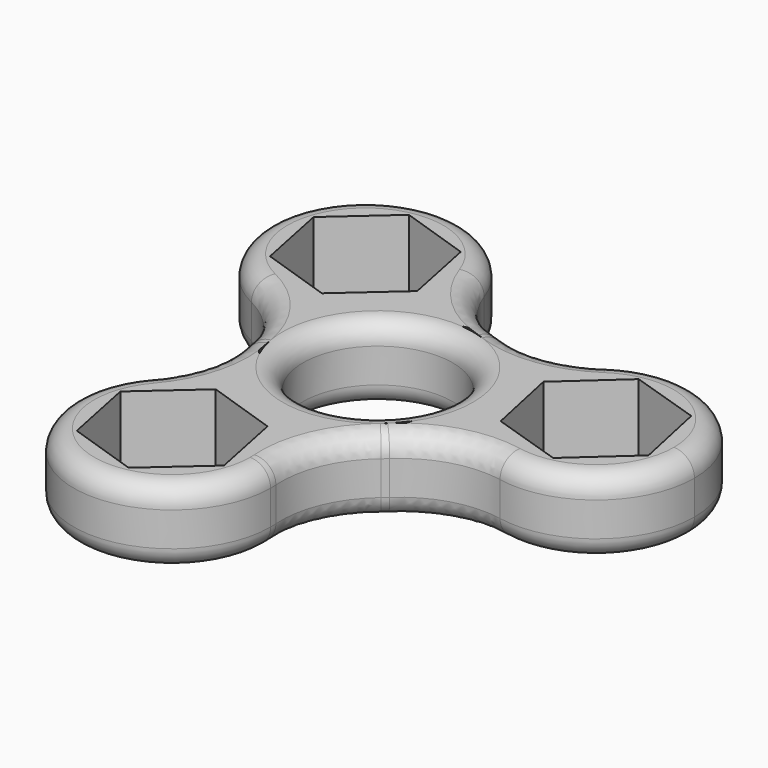
from build123d import *

# Parameters (mm, degrees)
F0_R     = 10.95
F1_DEPTH = 11
F2_R     = 15
F3_R     = 3
F4_R     = 3
F5_R     = 2.99999


# Not quite as in the source:
# - a fillet or chamfer is up to 0.001 mm smaller than in the source, because OpenCascade refuses the exact size


with BuildPart() as f1:
    # F0 (on Top) → F1 (new body)
    with BuildSketch(Plane.XY):
        with BuildLine():
            ThreePointArc((16.654712117, -4.1714415358), (16.9775112004, -2.2849104924), (17.0855701569, -0.3740149201))
            ThreePointArc((17.0855701569, -0.3740149201), (16.2517047433, 4.8769569892), (13.8321535207, 9.6112794751))
            ThreePointArc((13.8321535207, 9.6112794751), (13.447376375, 2.3521052012), (16.654712117, -4.1714415358))
        make_face()
        with BuildLine():
            ThreePointArc((13.8321535207, 9.6112794751), (16.2517047433, 4.8769569892), (17.0855701569, -0.3740149201))
            ThreePointArc((17.0855701569, -0.3740149201), (16.9775112004, -2.2849104924), (16.654712117, -4.1714415358))
            ThreePointArc((16.654712117, -4.1714415358), (32.5885679794, -8.2650064174), (41.9781924859, 5.2435089603))
            ThreePointArc((41.9781924859, 5.2435089603), (29.7762969315, 19.4849706892), (13.8321535207, 9.6112794751))
        make_face()
        Polygon((25.2852360408, 15.9143511546), (35.6669746396, 12.5543654899), (37.948010997, 1.8835232956), (29.8473087557, -5.4273332341), (19.4655701569, -2.0673475694), (17.1845337995, 8.6034946249), align=None, mode=Mode.SUBTRACT)
        with BuildLine():
            ThreePointArc((16.654712117, -4.1714415358), (13.447376375, 2.3521052012), (13.8321535207, 9.6112794751))
            ThreePointArc((13.8321535207, 9.6112794751), (5.4932428297, 15.7069627719), (-4.835332905, 15.8306949739))
            ThreePointArc((-4.835332905, 15.8306949739), (-8.8812222309, 9.7912873743), (-15.3602401355, 6.4949270203))
            ThreePointArc((-15.3602401355, 6.4949270203), (-16.4698013785, -3.7746231263), (-11.4126687413, -12.7812981985))
            ThreePointArc((-11.4126687413, -12.7812981985), (-4.1594436733, -13.2654373359), (1.9347970856, -17.2282512558))
            ThreePointArc((1.9347970856, -17.2282512558), (11.3832690194, -13.054384406), (16.654712117, -4.1714415358))
        make_face()
        with Locations((0.1355701569, -0.3740149201)):
            Circle(F0_R, mode=Mode.SUBTRACT)
        with BuildLine():
            ThreePointArc((-15.3602401355, 6.4949270203), (-8.8812222309, 9.7912873743), (-4.835332905, 15.8306949739))
            ThreePointArc((-4.835332905, 15.8306949739), (-11.1121287057, 12.3063545657), (-15.3602401355, 6.4949270203))
        make_face()
        with BuildLine():
            ThreePointArc((-15.3602401355, 6.4949270203), (-11.1121287057, 12.3063545657), (-4.835332905, 15.8306949739))
            ThreePointArc((-4.835332905, 15.8306949739), (-4.2348340755, 18.1680859941), (-4.0327792629, 20.5729081243))
            ThreePointArc((-4.0327792629, 20.5729081243), (-29.6731547282, 29.6075763776), (-15.3602401355, 6.4949270203))
        make_face()
        Polygon((-26.6131957882, 13.3378776512), (-28.7946677563, 24.0295183135), (-20.6261713186, 31.2645487867), (-10.2762029129, 27.8079385975), (-8.0947309448, 17.1162979351), (-16.2632273825, 9.881267462), align=None, mode=Mode.SUBTRACT)
        with BuildLine():
            ThreePointArc((5.6970575107, -26.938461845), (4.7236173339, -21.7316683693), (1.9347970856, -17.2282512558))
            ThreePointArc((1.9347970856, -17.2282512558), (-5.2221025159, -16.4549926121), (-11.4126687413, -12.7812981985))
            ThreePointArc((-11.4126687413, -12.7812981985), (-17.9024322709, -38.0421550924), (5.6970575107, -26.938461845))
        make_face()
        Polygon((1.6348588738, -30.3958113922), (-6.5341543893, -37.630258317), (-16.88387584, -34.1729087698), (-19.0645840278, -23.4811122978), (-10.8955707647, -16.2466653729), (-0.545849314, -19.7040149201), align=None, mode=Mode.SUBTRACT)
        with BuildLine():
            ThreePointArc((-11.4126687413, -12.7812981985), (-5.2221025159, -16.4549926121), (1.9347970856, -17.2282512558))
            ThreePointArc((1.9347970856, -17.2282512558), (-4.1594436733, -13.2654373359), (-11.4126687413, -12.7812981985))
        make_face()
    extrude(amount=F1_DEPTH)

    # F2
    f2_edges = [f1.edges().sort_by_distance(p)[0] for p in [
        (16.654712, -4.171442, 5.5),
        (1.934797, -17.228251, 5.5),
        (-11.412669, -12.781298, 5.5),
        (-15.36024, 6.494927, 5.5),
        (-4.835333, 15.830695, 5.5),
        (13.832154, 9.611279, 5.5),
    ]]
    fillet(f2_edges, radius=F2_R)

    # F3
    f3_edges = [f1.edges().sort_by_distance(p)[0] for p in [
        (-28.008176, 31.354529, 0),
        (41.685168, 8.134913, 0),
        (6.823784, -19.013919, 0),
    ]]
    fillet(f3_edges, radius=F3_R)

    # F4
    f4_edges = [f1.edges().sort_by_distance(p)[0] for p in [
        (-16.395705, -11.27792, 11),
        (-13.270281, -40.611486, 11),
        (6.823784, -19.013919, 11),
        (17.844267, -9.238567, 11),
        (41.685168, 8.134913, 11),
        (12.934093, 14.7381, 11),
        (-1.041851, 19.394442, 11),
    ]]
    fillet(f4_edges, radius=F4_R)

    # F5 (radius 3 in the source; OpenCascade refuses exactly that, so slightly less here)
    f5_edges = [f1.edges().sort_by_distance(p)[0] for p in [
        (-10.81443, -0.374015, 11),
        (-10.81443, -0.374015, 0),
    ]]
    fillet(f5_edges, radius=F5_R)


solid = f1.part
